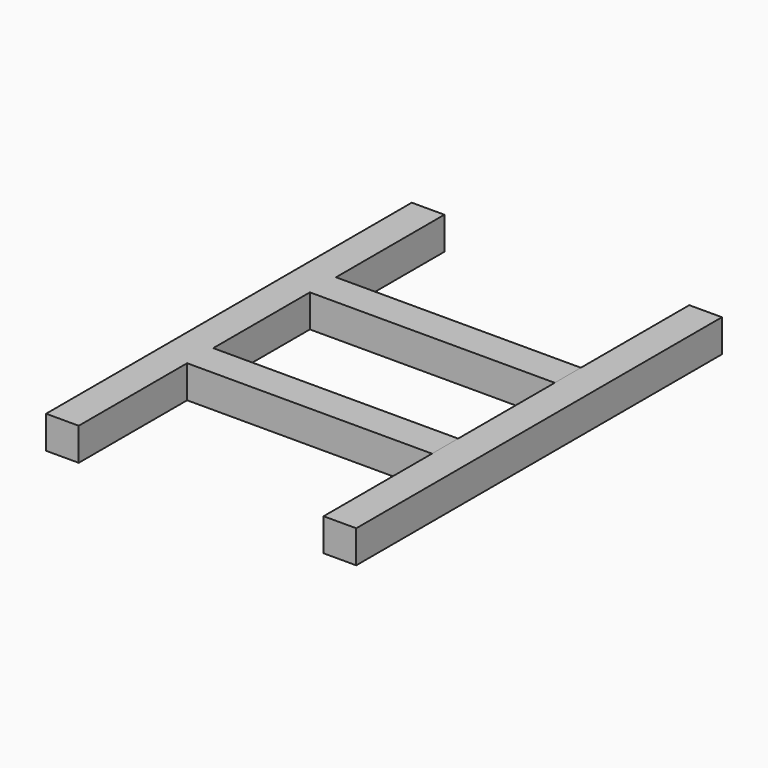
from build123d import *

# Parameters (mm, degrees)
F0_W     = 2
F0_H     = 2
F1_DEPTH = 28
F2_W     = 2
F2_H     = 2
F3_DEPTH = 15


# Not quite as in the source:
# - a feature names something its author has since deleted; it is built from what else it names


with BuildPart() as f1:
    # F0 (on Front) → F1 (new body)
    with BuildSketch(Plane.XZ):
        with Locations((-29.2174071148, 15.274727294)):
            Rectangle(F0_W, F0_H)
    extrude(amount=F1_DEPTH)

    # F2 (on face) → F3 (join)
    with BuildSketch(Plane.YZ.offset(-28.2174071148)):
        with Locations((-18.7, 15.274727294)):
            Rectangle(F2_W, F2_H)
        with Locations((-9.3, 15.274727294)):
            Rectangle(F2_W, F2_H)
    extrude(amount=F3_DEPTH)


with BuildPart() as f1b:
    # F0 (on Front) → F1, piece 2 (new body)
    with BuildSketch(Plane.XZ):
        with Locations((-12.2174071148, 15.274727294)):
            Rectangle(F0_W, F0_H)
    extrude(amount=F1_DEPTH)


solid = Compound([f1.part, f1b.part])
